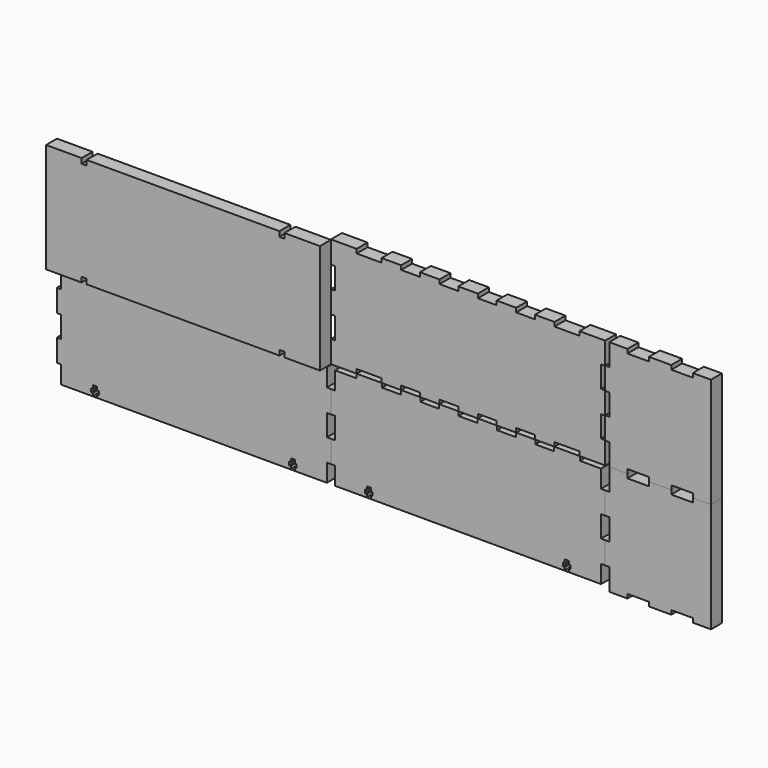
from build123d import *

# Parameters (mm, degrees)
F1_DEPTH = 10
F2_DEPTH = 10
F4_DEPTH = 25
F5_DEPTH = 25
F6_DEPTH = 10


# Not quite as in the source:
# - ends of sketch curves that miss each other by under 0.0002 mm in the source are joined
# - a feature of the source that left no trace in its solid (it failed there, or was rolled back) is left out
# - a feature names something its author has since deleted; it is built from what else it names


with BuildPart() as f1:
    # F0 (on Front) → F1 (new body)
    with BuildSketch(Plane.XZ):
        Polygon((-19.870002, 2e-06), (-20.130003, 2e-06), (-20.130003, -3.000001), (-35.630001, -3.000001), (-35.630001, -16), (-38.630001, -16), (-38.629996, -32.26), (-35.630001, -32.26), (-35.630001, -47.999997), (-38.630001, -47.999997), (-38.629996, -64.259998), (-35.630001, -64.259998), (-35.630001, -77.259998), (158.629981, -77.259998), (158.629981, -64.259998), (161.629985, -64.259998), (161.629985, -47.999997), (158.629981, -47.999997), (158.629981, -32.26), (161.629985, -32.26), (161.629985, -16), (158.629981, -16), (158.629981, -3.000001), (143.129994, -3.000001), (143.129994, -1e-06), (142.869993, 2e-06), (124.629985, -1e-06), (124.369984, 2e-06), (124.369984, -3.000001), (110.629991, -3.000001), (110.629991, -1e-06), (110.369989, 2e-06), (96.629987, -1e-06), (96.369995, 2e-06), (96.369995, -3.000001), (82.629993, -3.000001), (82.629993, -1e-06), (82.369992, 2e-06), (68.62999, -1e-06), (68.369989, 2e-06), (68.369989, -3.000001), (54.629995, -3.000001), (54.629995, -1e-06), (54.369994, 2e-06), (40.629992, -1e-06), (40.369991, 2e-06), (40.369991, -3.000001), (26.629994, -3.000001), (26.629994, -1e-06), (26.369997, 2e-06), (12.629995, -1e-06), (12.369998, 2e-06), (12.369998, -3.000001), (-1.370004, -3.000001), (-1.370004, -1e-06), (-1.630005, 2e-06), align=None)
    extrude(amount=F1_DEPTH)

    # F3 (on face) → F5 (cut)
    with BuildSketch(Plane.XZ.offset(10)):
        Polygon((-12.5035849761, -74.9435265806), (-12.5035849761, -77.0435265806), (-9.4035849761, -77.0435265806), (-9.4035849761, -74.9435265806), (-8.1535849761, -74.9435265806), (-8.1535849761, -72.4435265806), (-9.4035849761, -72.4435265806), (-9.4035849761, -69.9435265806), (-12.5035849761, -69.9435265806), (-12.5035849761, -72.4435265806), (-13.7535849761, -72.4435265806), (-13.7535849761, -74.9435265806), align=None)
        Polygon((131.9964070239, -74.9435265806), (131.9964070239, -77.0435265806), (135.0964040239, -77.0435265806), (135.0964040239, -74.9435265806), (136.3464040239, -74.9435265806), (136.3464040239, -72.4435265806), (135.0964040239, -72.4435265806), (135.0964040239, -69.9435265806), (131.9964070239, -69.9435265806), (131.9964070239, -72.4435265806), (130.7464060239, -72.4435265806), (130.7464060239, -74.9435265806), align=None)
    extrude(amount=-F5_DEPTH, mode=Mode.SUBTRACT)


with BuildPart() as f1b:
    # F0 (on Front) → F1, piece 2 (new body)
    with BuildSketch(Plane.XZ):
        Polygon((164.629985, 64.259995), (161.629985, 64.259995), (161.629985, 63.999995), (161.629985, 48.259996), (161.629985, 47.999995), (164.629985, 47.999995), (164.629985, 32.259998), (161.629985, 32.259998), (161.629985, 31.999997), (161.629985, 16.259998), (161.629985, 15.999997), (164.629985, 15.999997), (164.629985, 2e-06), (177.889984, 2e-06), (177.889984, 2.999997), (193.629983, 2.999997), (193.629983, 2e-06), (209.889981, 2e-06), (209.889981, 2.999997), (225.62998, 2.999997), (225.62998, 2e-06), (238.889982, 2e-06), (238.889982, 80.259993), (225.62998, 80.259993), (225.62998, 77.259994), (209.889981, 77.259994), (209.889981, 80.259993), (193.629983, 80.259993), (193.629983, 77.259994), (177.889984, 77.259994), (177.889984, 80.259993), (164.629985, 80.259993), align=None)
    extrude(amount=F1_DEPTH)


with BuildPart() as f2:
    # F0 (on Front) → F2 (new body)
    with BuildSketch(Plane.XZ):
        Polygon((-201.629985, -1e-06), (-220.389984, -1e-06), (-220.389984, -3.000001), (-235.889982, -3.000001), (-235.889982, -16), (-238.889982, -16), (-238.889982, -32.26), (-235.889982, -32.26), (-235.889982, -47.999997), (-238.889982, -47.999997), (-238.889982, -64.259998), (-235.889982, -64.259998), (-235.889982, -77.259998), (-41.629999, -77.259998), (-41.629999, -64.259998), (-38.629996, -64.259998), (-38.629996, -47.999997), (-41.629999, -47.999997), (-41.629999, -32.26), (-38.629996, -32.26), (-38.629996, -16), (-41.629999, -16), (-41.629999, -3.000001), (-57.129987, -3.000001), (-57.129987, -1e-06), (-75.889997, -1e-06), (-75.889997, -3.000001), (-89.62999, -3.000001), (-89.62999, -1e-06), (-103.889986, -1e-06), (-103.889986, -3.000001), (-117.629988, -3.000001), (-117.629988, -1e-06), (-131.889992, -1e-06), (-131.889992, -3.000001), (-145.629985, -3.000001), (-145.629985, -1e-06), (-159.889989, -1e-06), (-159.889989, -3.000001), (-173.629987, -3.000001), (-173.629987, -1e-06), (-187.889983, -1e-06), (-187.889983, -3.000001), (-201.629985, -3.000001), align=None)
    extrude(amount=F2_DEPTH)

    # F3 (on face) → F4 (cut)
    with BuildSketch(Plane.XZ.offset(10)):
        Polygon((-212.5035809761, -74.9435265806), (-212.5035809761, -77.0435265806), (-209.4035819761, -77.0435265806), (-209.4035819761, -74.9435265806), (-208.1535819761, -74.9435265806), (-208.1535819761, -72.4435265806), (-209.4035819761, -72.4435265806), (-209.4035819761, -69.9435265806), (-212.5035809761, -69.9435265806), (-212.5035809761, -72.4435265806), (-213.7535819761, -72.4435265806), (-213.7535819761, -74.9435265806), align=None)
        Polygon((-68.0035899761, -74.9435265806), (-68.0035899761, -77.0435265806), (-64.9035929761, -77.0435265806), (-64.9035929761, -74.9435265806), (-63.6535929761, -74.9435265806), (-63.6535929761, -72.4435265806), (-64.9035929761, -72.4435265806), (-64.9035929761, -69.9435265806), (-68.0035899761, -69.9435265806), (-68.0035899761, -72.4435265806), (-69.2535899761, -72.4435265806), (-69.2535899761, -74.9435265806), align=None)
    extrude(amount=-F4_DEPTH, mode=Mode.SUBTRACT)

    # F3 (on face) → F6 (join)
    with BuildSketch(Plane.XZ.offset(10)):
        Polygon((-238.7035809761, -0.0435265806), (-235.7035809761, -0.0435265806), (-220.2035829761, -0.0435265806), (-212.8035819761, -0.0435325806), (-212.8035819761, 3.6564674194), (-209.1035829761, 3.6564674194), (-209.1035829761, -0.0435325806), (-201.7035849761, -0.0435325806), (-187.7035819761, -0.0435265806), (-173.7035829761, -0.0435325806), (-159.7035879761, -0.0435265806), (-145.7035849761, -0.0435325806), (-131.7035909761, -0.0435265806), (-117.7035879761, -0.0435325806), (-103.7035849761, -0.0435265806), (-89.7035899761, -0.0435325806), (-75.7035959761, -0.0435265806), (-68.3035889761, -0.0435325806), (-68.3035889761, 3.6564674194), (-64.6035939761, 3.6564674194), (-64.6035939761, -0.0435325806), (-57.2035869761, -0.0435325806), (-41.7035989761, -0.0435265806), (-38.7035959761, -0.0435265806), (-38.7035959761, 2.9564674194), (-38.7035959761, 15.9564664194), (-38.7035959761, 31.9564654194), (-38.7035959761, 38.1064654194), (-38.7035959761, 41.8064644194), (-38.7035959761, 47.9564624194), (-38.7035959761, 63.9564624194), (-38.7035959761, 76.9564634194), (-38.7035959761, 79.9564664194), (-57.2035869761, 79.9564664194), (-64.6035939761, 79.9564664194), (-64.6035939761, 76.2564634194), (-68.3035889761, 76.2564634194), (-68.3035889761, 79.9564664194), (-75.7035959761, 79.9564664194), (-89.7035899761, 79.9564664194), (-103.7035849761, 79.9564664194), (-117.7035879761, 79.9564664194), (-131.7035909761, 79.9564664194), (-145.7035849761, 79.9564664194), (-159.7035879761, 79.9564664194), (-173.7035829761, 79.9564664194), (-187.7035819761, 79.9564664194), (-201.7035849761, 79.9564664194), (-209.1035829761, 79.9564664194), (-209.1035829761, 76.2564634194), (-212.8035819761, 76.2564634194), (-212.8035819761, 79.9564664194), (-220.2035829761, 79.9564664194), (-238.7035809761, 79.9564664194), (-238.7035809761, 76.9564634194), (-238.7035809761, 63.9564624194), (-238.7035809761, 47.9564624194), (-238.7035809761, 41.8064644194), (-238.7035809761, 38.1064654194), (-238.7035809761, 31.9564654194), (-238.7035809761, 15.9564664194), (-238.7035809761, 2.9564674194), align=None)
    extrude(amount=F6_DEPTH)


with BuildPart() as f2b:
    # F0 (on Front) → F2, piece 2 (new body)
    with BuildSketch(Plane.XZ):
        Polygon((-19.870002, 80.259993), (-38.630001, 80.259993), (-38.630001, 63.999995), (-35.630001, 63.999995), (-35.630001, 48.259996), (-38.630001, 48.259996), (-38.630001, 31.999997), (-35.630001, 31.999997), (-35.630001, 16.259998), (-38.630001, 16.259998), (-38.630001, 2e-06), (-20.130003, 2e-06), (-19.870002, 2e-06), (-19.870002, 2.999997), (-1.630005, 2.999997), (-1.630005, 2e-06), (-1.370004, 2e-06), (12.369998, 2e-06), (12.629995, 2e-06), (12.629995, 2.999997), (26.369997, 2.999997), (26.369997, 2e-06), (26.629994, 2e-06), (40.369991, 2e-06), (40.629992, 2e-06), (40.629992, 2.999997), (54.369994, 2.999997), (54.369994, 2e-06), (54.629995, 2e-06), (68.369989, 2e-06), (68.62999, 2e-06), (68.62999, 2.999997), (82.369992, 2.999997), (82.369992, 2e-06), (82.629993, 2e-06), (96.369995, 2e-06), (96.629987, 2e-06), (96.629987, 2.999997), (110.369989, 2.999997), (110.369989, 2e-06), (110.629991, 2e-06), (124.369984, 2e-06), (124.629985, 2e-06), (124.629985, 2.999997), (142.869993, 2.999997), (142.869993, 2e-06), (143.129994, 2e-06), (161.629985, 2e-06), (161.629985, 15.999997), (161.629985, 16.259998), (158.629981, 16.259998), (158.629981, 31.999997), (161.629985, 31.999997), (161.629985, 32.259998), (161.629985, 47.999995), (161.629985, 48.259996), (158.629981, 48.259996), (158.629981, 63.999995), (161.629985, 63.999995), (161.629985, 64.259995), (161.629985, 80.259993), (142.869993, 80.259993), (142.869993, 77.259994), (124.629985, 77.259994), (124.629985, 80.259993), (110.369989, 80.259993), (110.369989, 77.259994), (96.629987, 77.259994), (96.629987, 80.259993), (82.369992, 80.259993), (82.369992, 77.259994), (68.62999, 77.259994), (68.62999, 80.259993), (54.369994, 80.259993), (54.369994, 77.259994), (40.629992, 77.259994), (40.629992, 80.259993), (26.369997, 80.259993), (26.369997, 77.259994), (12.629995, 77.259994), (12.629995, 80.259993), (-1.630005, 80.259993), (-1.630005, 77.259994), (-19.870002, 77.259994), align=None)
    extrude(amount=F2_DEPTH)


with BuildPart() as f2c:
    # F0 (on Front) → F2, piece 3 (new body)
    with BuildSketch(Plane.XZ):
        Polygon((161.629985, -47.999997), (161.629985, -64.259998), (164.629985, -64.259998), (164.629985, -80.259993), (177.889984, -80.259993), (177.889984, -77.259998), (193.629983, -77.259998), (193.629983, -80.259993), (209.889981, -80.259993), (209.889981, -77.259998), (225.62998, -77.259998), (225.62998, -80.259993), (238.889982, -80.259993), (238.889982, -1e-06), (225.62998, 2e-06), (225.62998, -3.000001), (209.889981, -3.000001), (209.889981, -1e-06), (193.629983, 2e-06), (193.629983, -3.000001), (177.889984, -3.000001), (177.889984, -1e-06), (164.629985, 2e-06), (164.629985, -16), (161.629985, -16), (161.629985, -32.26), (164.629985, -32.26), (164.629985, -47.999997), align=None)
    extrude(amount=F2_DEPTH)


solid = Compound([f1.part, f1b.part, f2.part, f2b.part, f2c.part])
